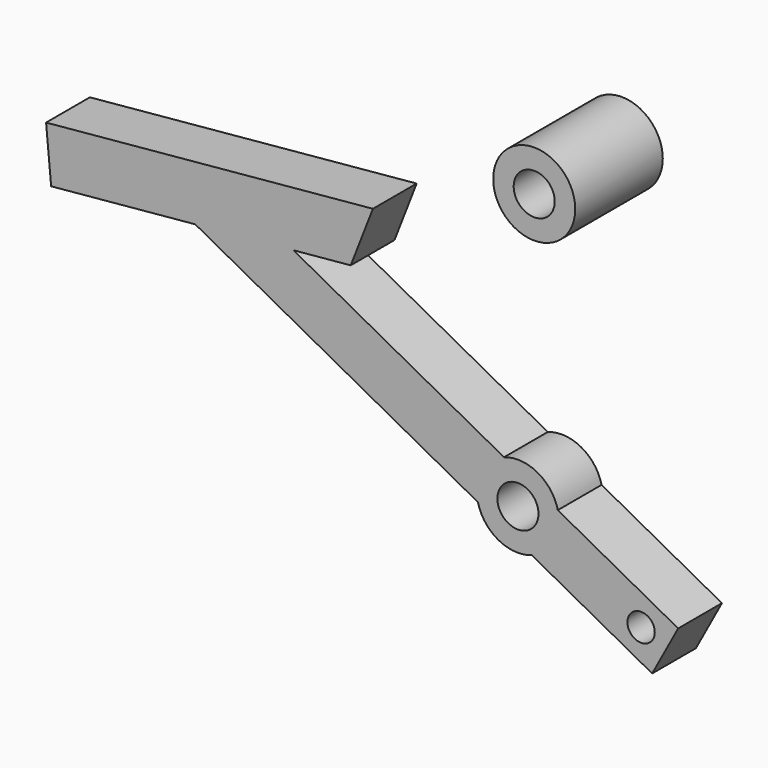
from build123d import *

# Parameters (mm, degrees)
F0_R     = 4.7625
F0_R_2   = 3.175
F1_DEPTH = 12.7
F0_R_3   = 9.525
F2_DEPTH = 25.4


# Not quite as in the source:
# - a feature names something its author has since deleted; it is built from what else it names


with BuildPart() as f1:
    # F0 (on Front) → F1 (new body)
    with BuildSketch(Plane.XZ):
        with BuildLine():
            ThreePointArc((3.2280459011, -8.9613249389), (7.7933549325, -5.4762435935), (9.525, 0))
            ThreePointArc((9.525, 0), (9.459652863, 1.1138189762), (9.264508092, 2.2123550376))
            ThreePointArc((9.264508092, 2.2123550376), (4.5273466432, 8.3802599824), (-3.2280459011, 8.9613249389))
            ThreePointArc((-3.2280459011, 8.9613249389), (-8.3802599824, 4.5273466432), (-9.264508092, -2.2123550376))
            ThreePointArc((-9.264508092, -2.2123550376), (-4.5273466432, -8.3802599824), (3.2280459011, -8.9613249389))
        make_face()
        Circle(F0_R, mode=Mode.SUBTRACT)
        with BuildLine():
            ThreePointArc((9.264508092, 2.2123550376), (9.459652863, 1.1138189762), (9.525, 0))
            ThreePointArc((9.525, 0), (7.7933549325, -5.4762435935), (3.2280459011, -8.9613249389))
            Line((3.2280459011, -8.9613249389), (31.1622458424, -24.0524804162))
            Line((31.1622458424, -24.0524804162), (37.1987080333, -12.8788004396))
            Line((37.1987080333, -12.8788004396), (9.264508092, 2.2123550376))
        make_face()
        with Locations((28.5936369496, -15.4474093325)):
            Circle(F0_R_2, mode=Mode.SUBTRACT)
        with BuildLine():
            ThreePointArc((-9.264508092, -2.2123550376), (-8.3802599824, 4.5273466432), (-3.2280459011, 8.9613249389))
            Line((-3.2280459011, 8.9613249389), (-52.1128957984, 35.3708470241))
            Line((-52.1128957984, 35.3708470241), (-74.9098779541, 33.251860334))
            Line((-74.9098779541, 33.251860334), (-9.264508092, -2.2123550376))
        make_face()
        Polygon((-74.9098779541, 33.251860334), (-52.1128957984, 35.3708470241), (-38.8146562076, 36.6069225934), (-33.6673133028, 49.8401142349), (-109.5402561535, 42.787700238), (-108.3648538207, 30.1422097629), align=None)
    extrude(amount=F1_DEPTH)


with BuildPart() as f2:
    # F0 (on Front) → F2 (new body)
    with BuildSketch(Plane.XZ):
        with Locations((13.9434637961, 73.5037211458)):
            Circle(F0_R_3)
        with Locations((13.9434637961, 73.5037211458)):
            Circle(F0_R, mode=Mode.SUBTRACT)
    extrude(amount=F2_DEPTH)


solid = Compound([f1.part, f2.part])
